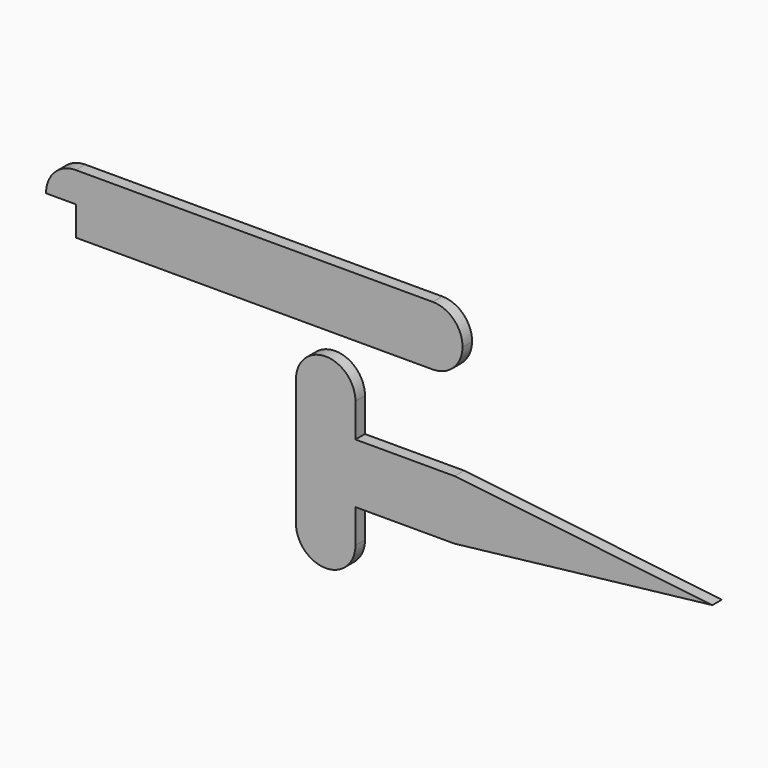
from build123d import *

# Parameters (mm, degrees)
F0_W     = 15
F0_H     = 15
F0_R     = 1.5
F1_DEPTH = 3


# Not quite as in the source:
# - a feature names something its author has since deleted; it is built from what else it names


with BuildPart() as f1:
    # F0 (on Front) → F1 (new body)
    with BuildSketch(Plane.XZ):
        with Locations((-7.5, 7.5)):
            Rectangle(F0_W, F0_H)
        with BuildLine():
            Line((-15, 15), (0, 15))
            Line((0, 15), (0, 23.5))
            ThreePointArc((0, 23.5), (-7.5, 31), (-15, 23.5))
            Line((-15, 23.5), (-15, 15))
        make_face()
        with Locations((-7.5, 23.5)):
            Circle(F0_R, mode=Mode.SUBTRACT)
        with Locations((-7.5, 23.5)):
            Circle(F0_R)
        with BuildLine():
            Line((0, -8.5), (0, 0))
            Line((0, 0), (-15, 0))
            Line((-15, 0), (-15, -8.5))
            ThreePointArc((-15, -8.5), (-7.5, -16), (0, -8.5))
        make_face()
        with Locations((-7.5, -8.5)):
            Circle(F0_R, mode=Mode.SUBTRACT)
        Polygon((0, 15), (0, 0), (25, 0), (90, 7.5), (25, 15), align=None)
        with Locations((-7.5, -8.5)):
            Circle(F0_R)
    extrude(amount=F1_DEPTH)


with BuildPart() as f1b:
    # F0 (on Front) → F1, piece 2 (new body)
    with BuildSketch(Plane.XZ):
        with BuildLine():
            Line((-70.5063530058, 44.2742461503), (-70.5063530058, 36.8742461503))
            Line((-70.5063530058, 36.8742461503), (19.4936469942, 36.8742461503))
            Line((19.4936469942, 36.8742461503), (19.4936469942, 42.8742461503))
            ThreePointArc((19.4936469942, 42.8742461503), (18.4689519176, 43.2788010352), (17.9969840395, 44.2742461503))
            Line((17.9969840395, 44.2742461503), (-59.8173476756, 44.2742461503))
            Line((-59.8173476756, 44.2742461503), (-70.5063530058, 44.2742461503))
        make_face()
        with BuildLine():
            Line((-70.5063530058, 51.8742461503), (-70.5063530058, 44.2742461503))
            Line((-70.5063530058, 44.2742461503), (-59.8173476756, 44.2742461503))
            Line((-59.8173476756, 44.2742461503), (17.9969840395, 44.2742461503))
            ThreePointArc((17.9969840395, 44.2742461503), (18.3982018792, 45.3989412269), (19.4936469942, 45.8742461503))
            Line((19.4936469942, 45.8742461503), (19.4936469942, 51.8742461503))
            Line((19.4936469942, 51.8742461503), (-70.5063530058, 51.8742461503))
        make_face()
        with BuildLine():
            Line((19.4936469942, 42.8742461503), (19.4936469942, 36.8742461503))
            ThreePointArc((19.4936469942, 36.8742461503), (24.7614738707, 39.0357070242), (26.9929802979, 44.2742461503))
            Line((26.9929802979, 44.2742461503), (20.9903099489, 44.2742461503))
            ThreePointArc((20.9903099489, 44.2742461503), (20.5183420708, 43.2788010352), (19.4936469942, 42.8742461503))
        make_face()
        with BuildLine():
            Line((20.9903099489, 44.2742461503), (26.9929802979, 44.2742461503))
            ThreePointArc((26.9929802979, 44.2742461503), (24.8321861202, 49.6420730267), (19.4936469942, 51.8742461503))
            Line((19.4936469942, 51.8742461503), (19.4936469942, 45.8742461503))
            ThreePointArc((19.4936469942, 45.8742461503), (20.554307166, 45.434906322), (20.9936469942, 44.3742461503))
            ThreePointArc((20.9936469942, 44.3742461503), (20.9928125008, 44.3242183183), (20.9903099489, 44.2742461503))
        make_face()
        with BuildLine():
            Line((19.4936469942, 45.8742461503), (19.4936469942, 44.2742461503))
            Line((19.4936469942, 44.2742461503), (20.9903099489, 44.2742461503))
            ThreePointArc((20.9903099489, 44.2742461503), (20.9928125008, 44.3242183183), (20.9936469942, 44.3742461503))
            ThreePointArc((20.9936469942, 44.3742461503), (20.554307166, 45.434906322), (19.4936469942, 45.8742461503))
        make_face()
        with BuildLine():
            Line((17.9969840395, 44.2742461503), (19.4936469942, 44.2742461503))
            Line((19.4936469942, 44.2742461503), (19.4936469942, 45.8742461503))
            ThreePointArc((19.4936469942, 45.8742461503), (18.3982018792, 45.3989412269), (17.9969840395, 44.2742461503))
        make_face()
        with BuildLine():
            Line((19.4936469942, 44.2742461503), (19.4936469942, 42.8742461503))
            ThreePointArc((19.4936469942, 42.8742461503), (20.5183420708, 43.2788010352), (20.9903099489, 44.2742461503))
            Line((20.9903099489, 44.2742461503), (19.4936469942, 44.2742461503))
        make_face()
        with BuildLine():
            ThreePointArc((17.9969840395, 44.2742461503), (18.4689519176, 43.2788010352), (19.4936469942, 42.8742461503))
            Line((19.4936469942, 42.8742461503), (19.4936469942, 44.2742461503))
            Line((19.4936469942, 44.2742461503), (17.9969840395, 44.2742461503))
        make_face()
        with BuildLine():
            Line((-78.0056863095, 44.2742461503), (-70.5063530058, 44.2742461503))
            Line((-70.5063530058, 44.2742461503), (-70.5063530058, 51.8742461503))
            ThreePointArc((-70.5063530058, 51.8742461503), (-75.8448921318, 49.6420730267), (-78.0056863095, 44.2742461503))
        make_face()
    extrude(amount=F1_DEPTH)


solid = Compound([f1.part, f1b.part])
